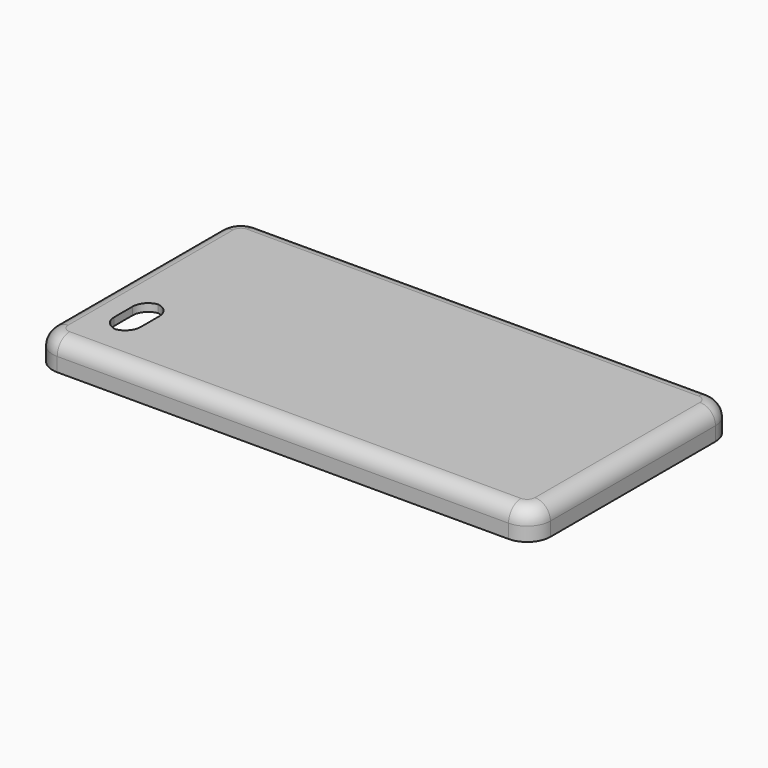
from build123d import *

# Parameters (mm, degrees)
F0_W        = 163.068
F0_H        = 82.804
F1_DEPTH    = 9.652
F2_R        = 7.62
F3_R        = 5.08
F4_T        = -2.54
F6_W        = 8.6941672489
F6_H        = 17.6881290972
F7_DEPTH    = 25.4
F8_T1_DEPTH = 2.54


# Not quite as in the source:
# - a fillet or chamfer that OpenCascade refuses, or shapes differently, is made with other operations: its cross-section is extruded or revolved along the edge and cut away or added


with BuildPart() as f1:
    # F0 (on Top) → F1 (new body)
    with BuildSketch(Plane.XY):
        with Locations((81.534, -41.402)):
            Rectangle(F0_W, F0_H)
    extrude(amount=F1_DEPTH)

    # F2
    f2_edges = [f1.edges().sort_by_distance(p)[0] for p in [
        (0, 0, 4.826),
        (163.068, 0, 4.826),
        (163.068, -82.804, 4.826),
        (0, -82.804, 4.826),
    ]]
    fillet(f2_edges, radius=F2_R)

    # F3
    f3_edges = [f1.edges().sort_by_distance(p)[0] for p in [
        (81.534, 0, 9.652),
        (160.836154, -2.231846, 9.652),
        (2.231846, -2.231846, 9.652),
        (163.068, -41.402, 9.652),
        (0, -41.402, 9.652),
        (160.836154, -80.572154, 9.652),
        (2.231846, -80.572154, 9.652),
        (81.534, -82.804, 9.652),
    ]]
    fillet(f3_edges, radius=F3_R)

    # F4
    f4_openings = [f1.faces().sort_by_distance(p)[0] for p in [
        (81.534, -41.402, 0),
    ]]
    offset(amount=F4_T, openings=f4_openings)

    # F6 (on face) → F7 (cut)
    with BuildSketch(Plane.XY.offset(9.652)):
        with Locations((15.8525095321, -60.5635698885)):
            Rectangle(F6_W, F6_H)
    extrude(amount=-F7_DEPTH, mode=Mode.SUBTRACT)

    # F8: fillet of radius 5.08 on 4 edges, made by hand

    # F8_s2 → F8_t1 (join)
    with BuildSketch(Plane.XY.offset(7.112)):
        with BuildLine():
            ThreePointArc((11.5054259077, -56.7995053399), (12.9933234592, -53.2074028914), (16.5854259077, -51.7195053399))
            Line((16.5854259077, -51.7195053399), (11.5054259077, -51.7195053399))
            Line((11.5054259077, -51.7195053399), (11.5054259077, -56.7995053399))
        make_face()
        with BuildLine():
            ThreePointArc((11.5054259077, -64.3276344371), (12.9933234592, -67.9197368855), (16.5854259077, -69.4076344371))
            Line((16.5854259077, -69.4076344371), (11.5054259077, -69.4076344371))
            Line((11.5054259077, -69.4076344371), (11.5054259077, -64.3276344371))
        make_face()
        with BuildLine():
            ThreePointArc((20.1995931566, -56.7995053399), (18.711695605, -53.2074028914), (15.1195931566, -51.7195053399))
            Line((15.1195931566, -51.7195053399), (20.1995931566, -51.7195053399))
            Line((20.1995931566, -51.7195053399), (20.1995931566, -56.7995053399))
        make_face()
        with BuildLine():
            ThreePointArc((15.1195931566, -69.4076344371), (18.711695605, -67.9197368855), (20.1995931566, -64.3276344371))
            Line((20.1995931566, -64.3276344371), (20.1995931566, -69.4076344371))
            Line((20.1995931566, -69.4076344371), (15.1195931566, -69.4076344371))
        make_face()
    extrude(amount=F8_T1_DEPTH)


solid = f1.part
